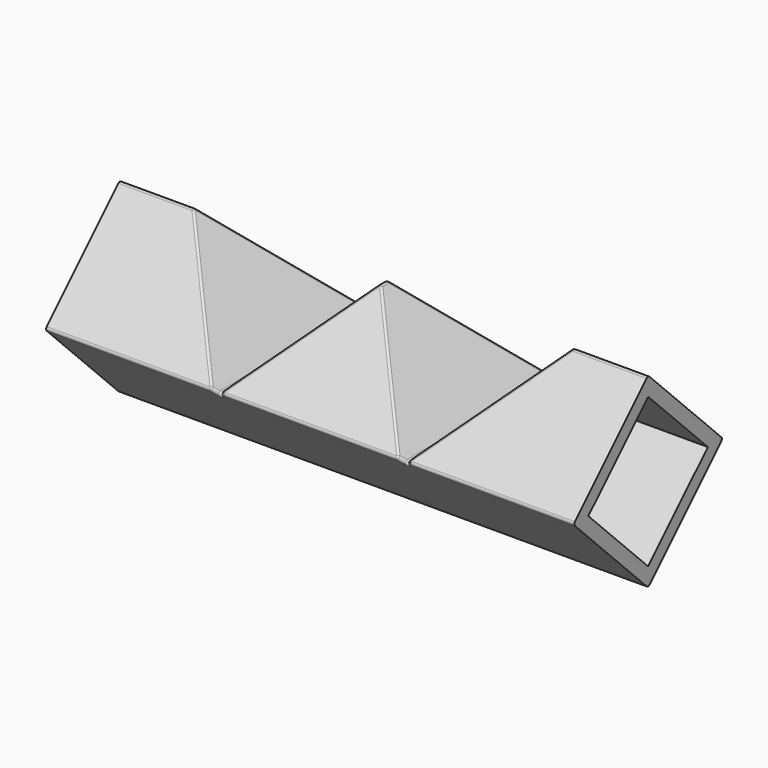
from build123d import *

# Parameters (mm, degrees)
F1_DEPTH      = 20
F4_DEPTH      = 7.0720678119
F4_DEPTH_BACK = 7.0720678119
F8_R          = 0.2
F9_T          = -1


# Not quite as in the source:
# - the program builds the solid bodies; features that only make, move or delete a surface that nothing else refers to are left out


with BuildPart() as f1:
    # F0 (on Right) → F1 (new body)
    with BuildSketch(Plane.YZ):
        Polygon((7.0710678119, 0), (0, 7.0710678119), (-7.0710678119, 0), (0, -7.0710678119), align=None)
    extrude(amount=F1_DEPTH)

    # F3 (on 3pt) → F4 (cut, two sides)
    with BuildSketch(Plane(origin=(0, 0, 0), x_dir=(-1, 0, 0), z_dir=(0, 1, 0))) as f4_sk:
        Polygon((0.2828427125, 7.0710678119), (-7.0710678119, 14.4249783362), (-14.4249783362, 7.0710678119), (-7.0710678119, -0.2828427125), align=None)
    extrude(amount=-F4_DEPTH, mode=Mode.SUBTRACT)
    extrude(f4_sk.sketch, amount=F4_DEPTH_BACK, mode=Mode.SUBTRACT)

    # F7: F1 across face


with BuildPart() as f1_1:
    add(f1.part)
    add(f1.part.mirror(Plane(origin=(0, 0, -0.0055104131), x_dir=(0, 1, 0), z_dir=(-1, 0, 0))))

    # F8
    f8_edges = [f1_1.edges().sort_by_distance(p)[0] for p in [
        (7.071068, 0, -0.282843),
        (3.394113, -3.676955, 3.394113),
        (3.394113, 3.676955, 3.394113),
        (0, 0, 6.788225),
        (6.929646, -6.929646, -0.141421),
        (6.929646, 6.929646, -0.141421),
        (7.212489, 6.929646, -0.141421),
        (7.212489, -6.929646, -0.141421),
        (10.889444, -3.535534, 3.535534),
        (10.889444, 3.535534, 3.535534),
        (17.212489, 0, 7.071068),
        (13.676955, 7.071068, 0),
        (13.676955, -7.071068, 0),
        (0, -7.071068, 0),
        (-13.676955, -7.071068, 0),
        (-7.212489, -6.929646, -0.141421),
        (-6.929646, -6.929646, -0.141421),
        (-10.889444, -3.535534, 3.535534),
        (-3.394113, -3.676955, 3.394113),
        (-3.394113, 3.676955, 3.394113),
        (-7.071068, 0, -0.282843),
        (-7.212489, 6.929646, -0.141421),
        (-6.929646, 6.929646, -0.141421),
        (-10.889444, 3.535534, 3.535534),
        (-17.212489, 0, 7.071068),
        (-13.676955, 7.071068, 0),
        (0, 7.071068, 0),
        (0, 0, -7.071068),
    ]]
    fillet(f8_edges, radius=F8_R)

    # F9
    f9_openings = [f1_1.faces().sort_by_distance(p)[0] for p in [
        (20, 0, 0),
        (-20, 0, 0),
    ]]
    offset(amount=F9_T, openings=f9_openings)


solid = f1_1.part
